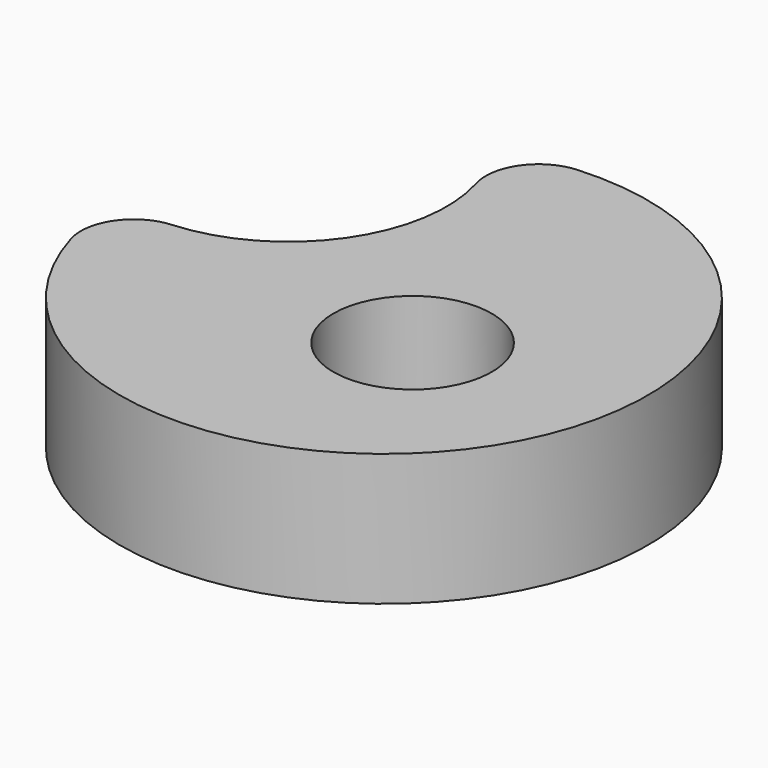
from build123d import *

# Parameters (mm, degrees)
F1_DEPTH = 25
F2_R     = 10


with BuildPart() as f1:
    # F0 (on Top) → F1 (new body)
    with BuildSketch(Plane.XY):
        with BuildLine():
            ThreePointArc((-16.4, 11.447270417), (-31.325290702, 0.2209930836), (-50, 0))
            ThreePointArc((-50, 0), (41, -28.6181760425), (-17.24, 46.9338087097))
            ThreePointArc((-17.24, 46.9338087097), (-11.0084011763, 29.3281056165), (-16.4, 11.447270417))
        make_face()
        with BuildLine():
            ThreePointArc((27.3, -8.5854528128), (7.8, -22.894540834), (0, 0))
            ThreePointArc((0, 0), (16.8, 5.7236352085), (27.3, -8.5854528128))
        make_face(mode=Mode.SUBTRACT)
    extrude(amount=F1_DEPTH)

    # F2
    f2_edges = [f1.edges().sort_by_distance(p)[0] for p in [
        (-50, 0, 12.5),
        (-17.24, 46.933809, 12.5),
    ]]
    fillet(f2_edges, radius=F2_R)


solid = f1.part
